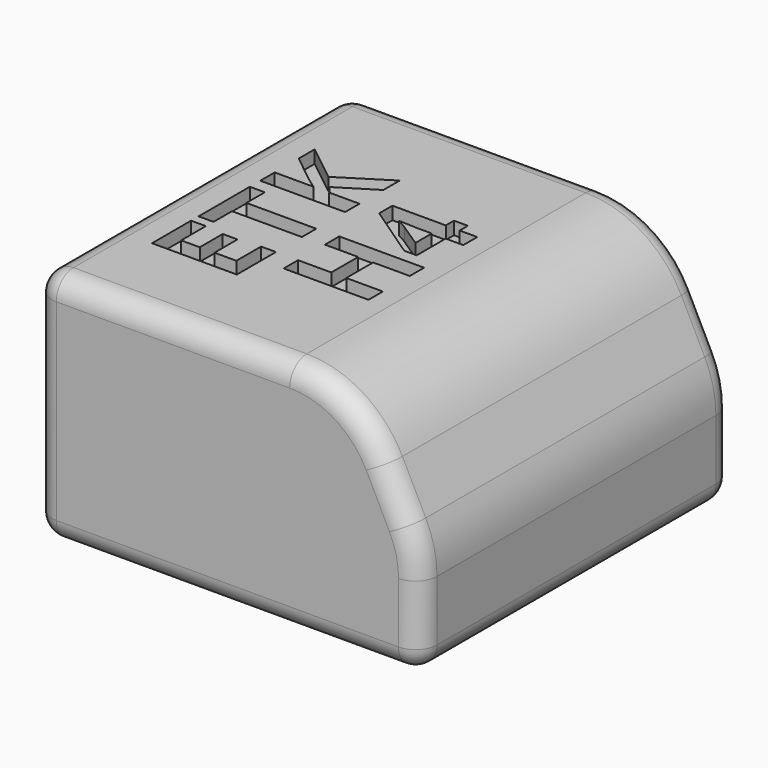
from build123d import *

# Parameters (mm, degrees)
F1_DEPTH     = 91.5
F2_R         = 5
F3_TEXT_SIZE = 27.7777777778
F4_TEXT_SIZE = 27.7777777778
F5_DEPTH     = 3


# Not quite as in the source:
# - Text() gives the source's letters only with a copy of the font that has no kerning and outlines rounded to 1/6400 em; it was checked with that copy


with BuildPart() as f1:
    # F0 (on Front) → F1 (new body)
    with BuildSketch(Plane.XZ):
        with BuildLine():
            Line((0, 55), (0, 0))
            Line((0, 0), (90, 0))
            Line((90, 0), (90, 19.0983005625))
            ThreePointArc((90, 19.0983005625), (89.3312247367, 24.8421235762), (87.360679775, 30.27864045))
            Line((87.360679775, 30.27864045), (81.9098300563, 41.1803398875))
            ThreePointArc((81.9098300563, 41.1803398875), (72.6924280842, 51.2662702088), (59.5491502813, 55))
            Line((59.5491502813, 55), (0, 55))
        make_face()
    extrude(amount=F1_DEPTH)

    # F2
    f2_edges = [f1.edges().sort_by_distance(p)[0] for p in [
        (29.774575, -91.5, 55),
        (0, -91.5, 27.5),
        (45, -91.5, 0),
        (29.774575, 0, 55),
        (45, 0, 0),
        (0, 0, 27.5),
        (0, -45.75, 0),
        (0, -45.75, 55),
        (90, -45.75, 0),
    ]]
    fillet(f2_edges, radius=F2_R)

    # F3 (on face) + F4 (on face) → F5 (cut)
    with BuildSketch(Plane.XY.offset(55)):
        with Locations(Location((30, -72.5), (0, 0, 90))):
            Text('ETK', F3_TEXT_SIZE, font='Open Sans', font_style=FontStyle.BOLD, text_align=(TextAlign.LEFT, TextAlign.BOTTOM))
    with BuildSketch(Plane.XY.offset(55)):
        with Locations(Location((55, -65.2821180556), (0, 0, 90))):
            Text('H4', F4_TEXT_SIZE, font='Open Sans', font_style=FontStyle.BOLD, text_align=(TextAlign.LEFT, TextAlign.BOTTOM))
    extrude(amount=-F5_DEPTH, mode=Mode.SUBTRACT)


solid = f1.part
